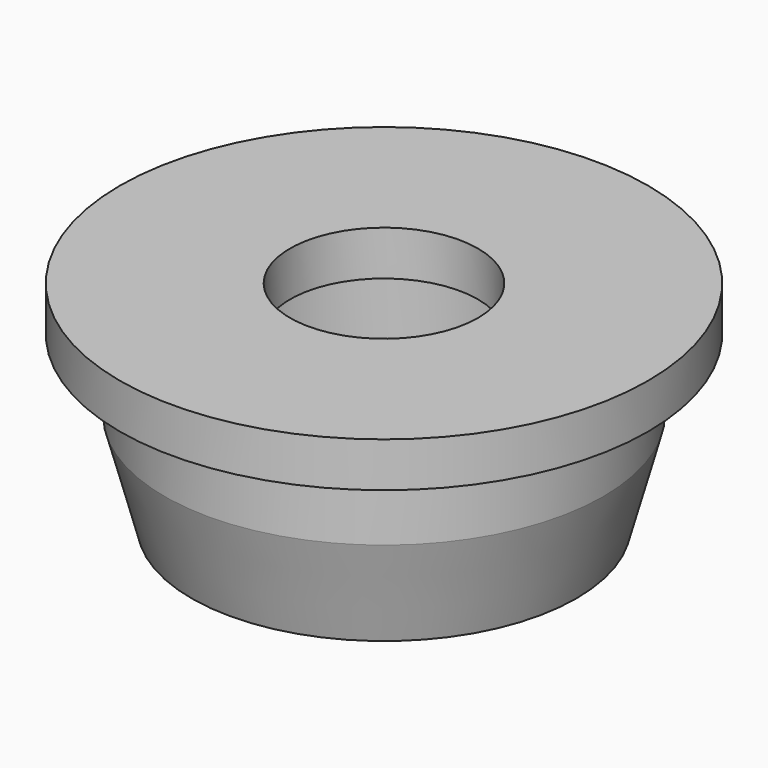
from build123d import *

# Parameters (mm, degrees)
F0_R     = 24.5
F0_R_2   = 15
F0_R_3   = 10.5
F1_DEPTH = 24
F2_SIZE2 = 3
F2_SIZE  = 11
F0_R_4   = 29.5
F3_DEPTH = 16
F4_DEPTH = 5
F5_DEPTH = 5


# Not quite as in the source:
# - a feature names something its author has since deleted; it is built from what else it names


with BuildPart() as f1:
    # F0 (on Top) → F1 (new body)
    with BuildSketch(Plane.XY):
        Circle(F0_R)
        Circle(F0_R_2, mode=Mode.SUBTRACT)
        Circle(F0_R_2)
        Circle(F0_R_3, mode=Mode.SUBTRACT)
        Circle(F0_R_3)
    extrude(amount=-F1_DEPTH)

    # F2
    f2_edges = [f1.edges().sort_by_distance(p)[0] for p in [
        (-24.5, 0, -24),
    ]]
    f2_side = f1.faces().sort_by_distance((-24.5, 0, -12))[0]
    chamfer(f2_edges, length=F2_SIZE, length2=F2_SIZE2, reference=f2_side)

    # F0 (on Top) → F3 (cut)
    with BuildSketch(Plane.XY):
        Circle(F0_R_4)
        Circle(F0_R, mode=Mode.SUBTRACT)
        Circle(F0_R_2)
        Circle(F0_R_3, mode=Mode.SUBTRACT)
        Circle(F0_R_3)
    extrude(amount=-F3_DEPTH, mode=Mode.SUBTRACT)

    # F0 (on Top) → F4 (join)
    with BuildSketch(Plane.XY):
        Circle(F0_R_2)
        Circle(F0_R_3, mode=Mode.SUBTRACT)
    extrude(amount=-F4_DEPTH)

    # F0 (on Top) → F5 (join)
    with BuildSketch(Plane.XY):
        Circle(F0_R_4)
        Circle(F0_R, mode=Mode.SUBTRACT)
    extrude(amount=-F5_DEPTH)


solid = f1.part
